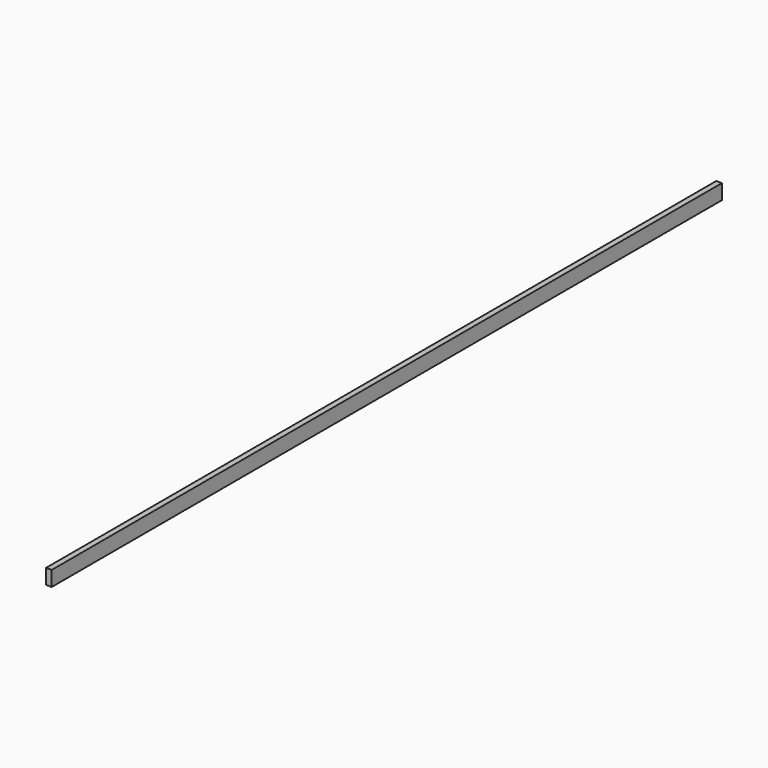
from build123d import *

# Parameters (mm, degrees)
F0_W     = 19.05
F0_H     = 50.8
F1_DEPTH = 2827.8666666667


# Not quite as in the source:
# - a length typed as a fraction of an inch, garbled in the dataset ("3 / 203.2 mm" for 3/8 in), is restored


with BuildPart() as f1:
    # F0 (on Front) → F1 (new body)
    with BuildSketch(Plane.XZ):
        with Locations((9.525, -25.4)):
            Rectangle(F0_W, F0_H)
    extrude(amount=-F1_DEPTH)


solid = f1.part
